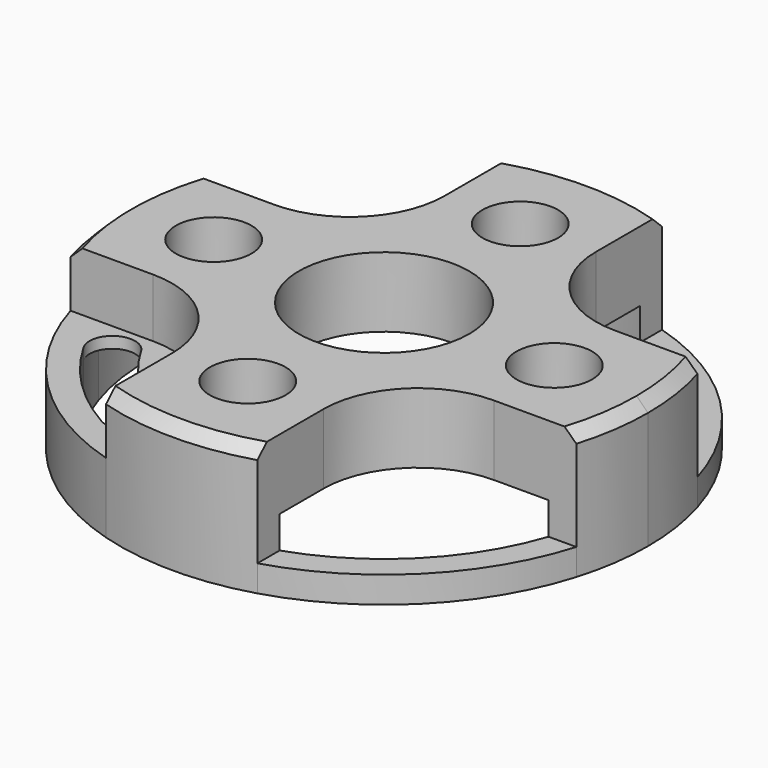
from build123d import *
from build123d import SkipClean  # not in build123d's __all__

# Parameters (mm, degrees)
F0_R     = 1
F0_R_2   = 2.25
F1_DEPTH = 3.4
F2_DEPTH = 0.7
F3_DEPTH = 1.85
F4_DEPTH = 1.55
F5_R     = 2.5
F6_SIZE  = 0.3
F8_DEPTH = 1.851


# Not quite as in the source:
# - after a boolean that leaves OpenCascade's solid faulty, fix() repairs it


with BuildPart() as f1:
    # F0 (on Top) → F1 (new body)
    with BuildSketch(Plane.XY):
        with BuildLine():
            Line((2, 5.9477411679), (2, 6.6821123157))
            ThreePointArc((2, 6.6821123157), (0, 6.975), (-2, 6.6821123157))
            Line((-2, 6.6821123157), (-2, 5.9477411679))
            ThreePointArc((-2, 5.9477411679), (0, 6.275), (2, 5.9477411679))
        make_face()
        with BuildLine():
            ThreePointArc((6.275, 0), (6.1926448642, 1.013298863), (5.9477411679, 2))
            Line((5.9477411679, 2), (2, 2))
            Line((2, 2), (2, 5.9477411679))
            ThreePointArc((2, 5.9477411679), (0, 6.275), (-2, 5.9477411679))
            Line((-2, 5.9477411679), (-2, 2))
            Line((-2, 2), (-5.9477411679, 2))
            ThreePointArc((-5.9477411679, 2), (-6.275, 0), (-5.9477411679, -2))
            Line((-5.9477411679, -2), (-2, -2))
            Line((-2, -2), (-2, -5.9477411679))
            ThreePointArc((-2, -5.9477411679), (0, -6.275), (2, -5.9477411679))
            Line((2, -5.9477411679), (2, -2))
            Line((2, -2), (5.9477411679, -2))
            ThreePointArc((5.9477411679, -2), (6.1926448642, -1.013298863), (6.275, 0))
        make_face()
        with Locations((0, -4.5)):
            Circle(F0_R, mode=Mode.SUBTRACT)
        with Locations((-4.5, 0)):
            Circle(F0_R, mode=Mode.SUBTRACT)
        Circle(F0_R_2, mode=Mode.SUBTRACT)
        with Locations((4.5, 0)):
            Circle(F0_R, mode=Mode.SUBTRACT)
        with Locations((0, 4.5)):
            Circle(F0_R, mode=Mode.SUBTRACT)
        with BuildLine():
            ThreePointArc((6.6821123157, -2), (6.9013896572, -1.0106660175), (6.975, 0))
            ThreePointArc((6.975, 0), (6.9013896572, 1.0106660175), (6.6821123157, 2))
            Line((6.6821123157, 2), (5.9477411679, 2))
            ThreePointArc((5.9477411679, 2), (6.1926448642, 1.013298863), (6.275, 0))
            ThreePointArc((6.275, 0), (6.1926448642, -1.013298863), (5.9477411679, -2))
            Line((5.9477411679, -2), (6.6821123157, -2))
        make_face()
        with BuildLine():
            Line((-5.9477411679, 2), (-6.6821123157, 2))
            ThreePointArc((-6.6821123157, 2), (-6.975, 0), (-6.6821123157, -2))
            Line((-6.6821123157, -2), (-5.9477411679, -2))
            ThreePointArc((-5.9477411679, -2), (-6.275, 0), (-5.9477411679, 2))
        make_face()
        with BuildLine():
            ThreePointArc((-2, -6.6821123157), (0, -6.975), (2, -6.6821123157))
            Line((2, -6.6821123157), (2, -5.9477411679))
            ThreePointArc((2, -5.9477411679), (0, -6.275), (-2, -5.9477411679))
            Line((-2, -5.9477411679), (-2, -6.6821123157))
        make_face()
    extrude(amount=F1_DEPTH)

    # F0 (on Top) → F2 (join)
    with BuildSketch(Plane.XY):
        with BuildLine():
            Line((-2, 5.9477411679), (-2, 6.6821123157))
            ThreePointArc((-2, 6.6821123157), (-4.9320697988, 4.9320697988), (-6.6821123157, 2))
            Line((-6.6821123157, 2), (-5.9477411679, 2))
            ThreePointArc((-5.9477411679, 2), (-4.4370950519, 4.4370950519), (-2, 5.9477411679))
        make_face()
        with BuildLine():
            Line((5.9477411679, 2), (6.6821123157, 2))
            ThreePointArc((6.6821123157, 2), (4.9320697988, 4.9320697988), (2, 6.6821123157))
            Line((2, 6.6821123157), (2, 5.9477411679))
            ThreePointArc((2, 5.9477411679), (4.4370950519, 4.4370950519), (5.9477411679, 2))
        make_face()
        with BuildLine():
            ThreePointArc((2, -6.6821123157), (4.9320697988, -4.9320697988), (6.6821123157, -2))
            Line((6.6821123157, -2), (5.9477411679, -2))
            ThreePointArc((5.9477411679, -2), (4.4370950519, -4.4370950519), (2, -5.9477411679))
            Line((2, -5.9477411679), (2, -6.6821123157))
        make_face()
    extrude(amount=F2_DEPTH)

    # F0 (on Top) → F3 (join, through all)
    with BuildSketch(Plane.XY):
        with BuildLine():
            ThreePointArc((-5.9477411679, -2), (-4.4370950519, -4.4370950519), (-2, -5.9477411679))
            Line((-2, -5.9477411679), (-2, -2))
            Line((-2, -2), (-5.9477411679, -2))
        make_face()
        with BuildLine():
            ThreePointArc((-6.6821123157, -2), (-4.9320697988, -4.9320697988), (-2, -6.6821123157))
            Line((-2, -6.6821123157), (-2, -5.9477411679))
            ThreePointArc((-2, -5.9477411679), (-4.4370950519, -4.4370950519), (-5.9477411679, -2))
            Line((-5.9477411679, -2), (-6.6821123157, -2))
        make_face()
    extrude(amount=F3_DEPTH)

    # F0 (on Top) → F4 (cut, through all)
    with BuildSketch(Plane.XY):
        with BuildLine():
            ThreePointArc((6.275, 0), (6.1926448642, 1.013298863), (5.9477411679, 2))
            Line((5.9477411679, 2), (2, 2))
            Line((2, 2), (2, 5.9477411679))
            ThreePointArc((2, 5.9477411679), (0, 6.275), (-2, 5.9477411679))
            Line((-2, 5.9477411679), (-2, 2))
            Line((-2, 2), (-5.9477411679, 2))
            ThreePointArc((-5.9477411679, 2), (-6.275, 0), (-5.9477411679, -2))
            Line((-5.9477411679, -2), (-2, -2))
            Line((-2, -2), (-2, -5.9477411679))
            ThreePointArc((-2, -5.9477411679), (0, -6.275), (2, -5.9477411679))
            Line((2, -5.9477411679), (2, -2))
            Line((2, -2), (5.9477411679, -2))
            ThreePointArc((5.9477411679, -2), (6.1926448642, -1.013298863), (6.275, 0))
        make_face()
        with Locations((0, -4.5)):
            Circle(F0_R, mode=Mode.SUBTRACT)
        with Locations((-4.5, 0)):
            Circle(F0_R, mode=Mode.SUBTRACT)
        Circle(F0_R_2, mode=Mode.SUBTRACT)
        with Locations((4.5, 0)):
            Circle(F0_R, mode=Mode.SUBTRACT)
        with Locations((0, 4.5)):
            Circle(F0_R, mode=Mode.SUBTRACT)
        with BuildLine():
            ThreePointArc((-5.9477411679, -2), (-4.4370950519, -4.4370950519), (-2, -5.9477411679))
            Line((-2, -5.9477411679), (-2, -2))
            Line((-2, -2), (-5.9477411679, -2))
        make_face()
    with SkipClean():  # cleaning this boolean's faces spoils the solid; the shape is the same uncleaned
        extrude(amount=F4_DEPTH, mode=Mode.SUBTRACT)

    # F5
    f5_edges = [f1.edges().sort_by_distance(p)[0] for p in [
        (-2, 2, 2.475),
        (-2, -2, 2.625),
        (2, -2, 2.475),
        (2, 2, 2.475),
    ]]
    fillet(f5_edges, radius=F5_R)

    # F6
    f6_edges = [f1.edges().sort_by_distance(p)[0] for p in [
        (0, -6.975, 3.4),
        (6.975, 0, 3.4),
        (0, 6.975, 3.4),
        (-6.975, 0, 3.4),
    ]]
    chamfer(f6_edges, length=F6_SIZE)

    # F7 (on face) → F8 (cut, through all)
    with BuildSketch(Plane.XY.offset(1.85)):
        with BuildLine():
            ThreePointArc((-5.4520938065, -3.106492898), (-4.777137974, -3.3894531711), (-4.330778064, -2.8094577205))
            ThreePointArc((-4.330778064, -2.8094577205), (-4.3507826134, -2.6558176305), (-4.4094623216, -2.512422543))
            ThreePointArc((-4.4094623216, -2.512422543), (-5.2278132415, -2.288141978), (-5.4520938065, -3.106492898))
        make_face()
        with BuildLine():
            ThreePointArc((-4.4094623216, -2.512422543), (-4.3507826134, -2.6558176305), (-4.330778064, -2.8094577205))
            ThreePointArc((-4.330778064, -2.8094577205), (-4.777137974, -3.3894531711), (-5.4520938065, -3.106492898))
            ThreePointArc((-5.4520938065, -3.106492898), (-4.4370950519, -4.4370950519), (-3.106492898, -5.4520938065))
            ThreePointArc((-3.106492898, -5.4520938065), (-3.3307734629, -4.6337428865), (-2.512422543, -4.4094623216))
            ThreePointArc((-2.512422543, -4.4094623216), (-3.5885669145, -3.5885669145), (-4.4094623216, -2.512422543))
        make_face()
        with BuildLine():
            ThreePointArc((-2.2094577205, -4.930778064), (-2.2906990548, -4.6292992974), (-2.512422543, -4.4094623216))
            ThreePointArc((-2.512422543, -4.4094623216), (-3.3307734629, -4.6337428865), (-3.106492898, -5.4520938065))
            ThreePointArc((-3.106492898, -5.4520938065), (-2.5079789538, -5.4495367298), (-2.2094577205, -4.930778064))
        make_face()
    extrude(amount=-F8_DEPTH, mode=Mode.SUBTRACT)

    add(f1.part.fix(), mode=Mode.REPLACE)


solid = f1.part
